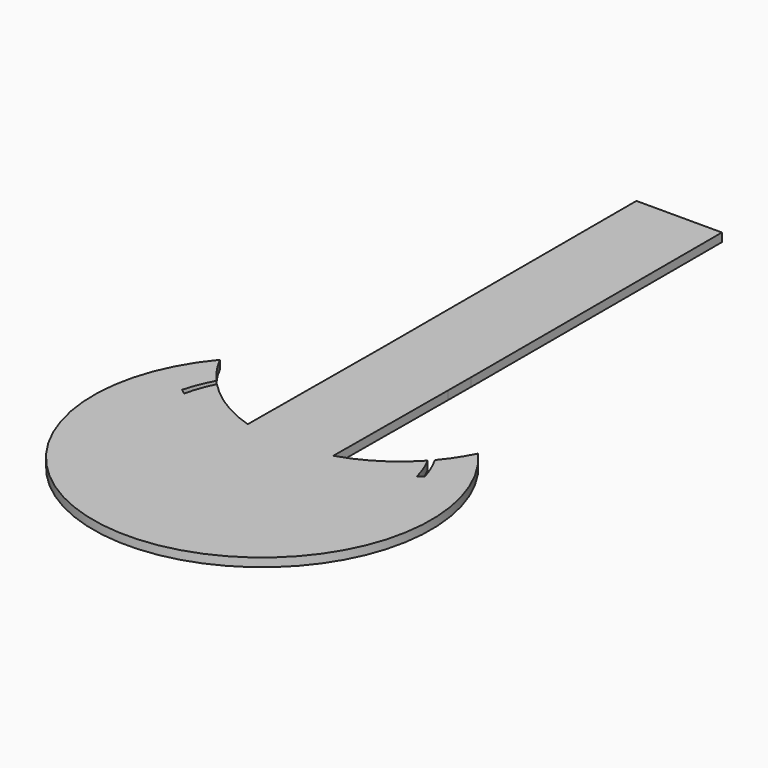
from build123d import *

# Parameters (mm, degrees)
F0_W     = 60
F0_H     = 220
F1_DEPTH = 6


# Not quite as in the source:
# - the program builds the solid bodies; features that only make, move or delete a surface that nothing else refers to are left out


with BuildPart() as f1:
    # F0 (on Top) → F1 (new body)
    with BuildSketch(Plane.XY):
        with Locations((4.8876879096, 45.2179194741)):
            Rectangle(F0_W, F0_H)
        with BuildLine():
            ThreePointArc((-79.4584430704, -175.2136584167), (-76.086405566, -164.9666401832), (-71.4764851469, -155.2136584167))
            ThreePointArc((-71.4764851469, -155.2136584167), (-79.1565485083, -145.3205641479), (-85.5490516624, -134.5505784994))
            ThreePointArc((-85.5490516624, -134.5505784994), (6.1468085688, -329.3233337338), (94.4628409087, -132.9949471034))
            ThreePointArc((94.4628409087, -132.9949471034), (88.2574232589, -143.8738017875), (80.7494829473, -153.8981481364))
            ThreePointArc((80.7494829473, -153.8981481364), (85.2254366965, -162.8589485125), (88.6456429035, -172.2734211397))
            ThreePointArc((88.6456429035, -172.2734211397), (75.2367314586, -249.2062042963), (5.6459887203, -284.6403764396))
            ThreePointArc((5.6459887203, -284.6403764396), (-63.9155377146, -250.9329661403), (-79.4584430704, -175.2136584167))
        make_face()
        with BuildLine():
            ThreePointArc((4.8876879096, -189.3289751767), (-10.6634233248, -188.2490297182), (-25.8614792361, -184.7816907769))
            ThreePointArc((-25.8614792361, -184.7816907769), (-48.9823809676, -174.2243385437), (-68.7229965841, -158.2136584167))
            ThreePointArc((-68.7229965841, -158.2136584167), (-72.9335538665, -167.9839691049), (-75.8560904631, -178.2136584167))
            ThreePointArc((-75.8560904631, -178.2136584167), (-59.2361153237, -247.9542245013), (5.5975931326, -278.5574984969))
            Line((5.5975931326, -278.5574984969), (4.8876879096, -189.3289751767))
        make_face()
        with BuildLine():
            ThreePointArc((78.0917461365, -156.8981481364), (57.9442467877, -173.7054474984), (34.1385207639, -184.7369682609))
            ThreePointArc((34.1385207639, -184.7369682609), (19.6828166371, -188.1140297879), (4.8876879096, -189.3289751767))
            Line((4.8876879096, -189.3289751767), (5.5975931326, -278.5574984969))
            ThreePointArc((5.5975931326, -278.5574984969), (70.4913174106, -246.4384867175), (85.2871903638, -175.5589515052))
            ThreePointArc((85.2871903638, -175.5589515052), (82.255170922, -166.010419768), (78.0917461365, -156.8981481364))
        make_face()
        with BuildLine():
            ThreePointArc((5.5975931326, -278.5574984969), (-59.2361153237, -247.9542245013), (-75.8560904631, -178.2136584167))
            Line((-75.8560904631, -178.2136584167), (-79.4584430704, -175.2136584167))
            ThreePointArc((-79.4584430704, -175.2136584167), (-63.9155377146, -250.9329661403), (5.6459887203, -284.6403764396))
            Line((5.6459887203, -284.6403764396), (5.5975931326, -278.5574984969))
        make_face()
        with BuildLine():
            ThreePointArc((85.2871903638, -175.5589515052), (70.4913174106, -246.4384867175), (5.5975931326, -278.5574984969))
            Line((5.5975931326, -278.5574984969), (5.6459887203, -284.6403764396))
            ThreePointArc((5.6459887203, -284.6403764396), (75.2367314586, -249.2062042963), (88.6456429035, -172.2734211397))
            Line((88.6456429035, -172.2734211397), (85.2871903638, -175.5589515052))
        make_face()
        with BuildLine():
            Line((34.7627821954, -84.7816907769), (-25.2371712536, -84.7816907769))
            Line((-25.2371712536, -84.7816907769), (-25.8614792361, -184.7816907769))
            ThreePointArc((-25.8614792361, -184.7816907769), (-10.6634233248, -188.2490297182), (4.8876879096, -189.3289751767))
            ThreePointArc((4.8876879096, -189.3289751767), (19.6828166371, -188.1140297879), (34.1385207639, -184.7369682609))
            Line((34.1385207639, -184.7369682609), (34.7627821954, -84.7816907769))
        make_face()
        Polygon((34.8876879096, -64.7820805259), (-25.1123120904, -64.7820805259), (-25.2371712536, -84.7816907769), (34.7627821954, -84.7816907769), align=None)
    extrude(amount=F1_DEPTH)


solid = f1.part
